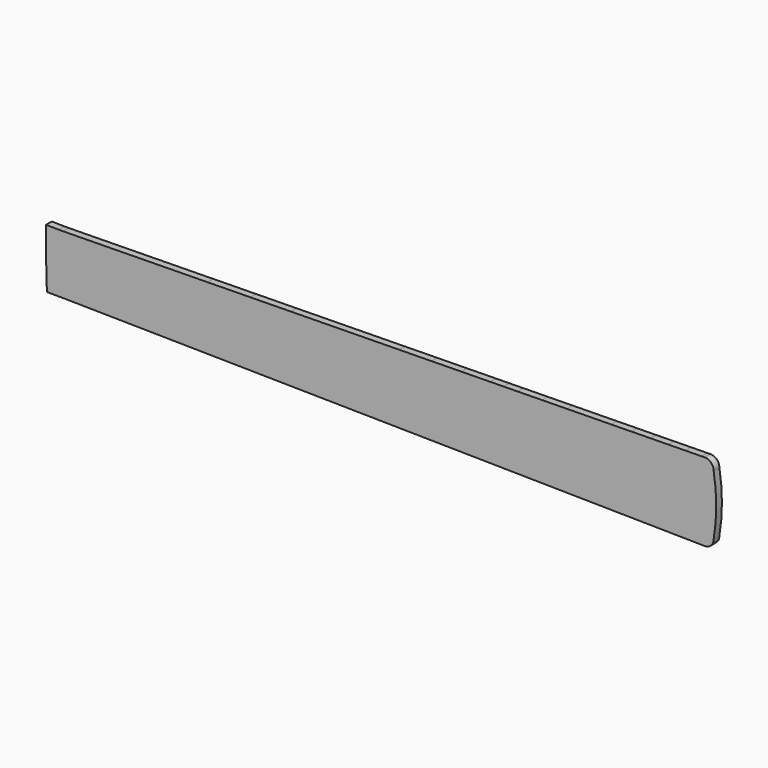
from build123d import *

# Parameters (mm, degrees)
F0_W     = 3.0600779591
F0_H     = 20.955
F1_DEPTH = 5.08


# Not quite as in the source:
# - a feature names something its author has since deleted; it is built from what else it names


with BuildPart() as f1:
    # F0 (on Front) → F1 (new body)
    with BuildSketch(Plane.XZ):
        with BuildLine():
            Line((211.1527612069, 54.1871569779), (194.9475612069, 53.9441942956))
            Line((194.9475612069, 53.9441942956), (194.9475612069, 27.6040292631))
            Line((194.9475612069, 27.6040292631), (199.8751612069, 27.6040292631))
            ThreePointArc((199.8751612069, 27.6040292631), (203.0501612069, 30.7790292631), (206.2251612069, 27.6040292631))
            Line((206.2251612069, 27.6040292631), (211.1527612069, 27.6040292631))
            Line((211.1527612069, 27.6040292631), (211.1527612069, 54.1871569779))
        make_face()
        with BuildLine():
            Line((35.1561612069, 27.6040292631), (25.4787612069, 27.6040292631))
            Line((25.4787612069, 27.6040292631), (25.4787612069, 3.8046848733))
            Line((25.4787612069, 3.8046848733), (51.1835612069, 3.4192950591))
            Line((51.1835612069, 3.4192950591), (51.1835612069, 27.6040292631))
            Line((51.1835612069, 27.6040292631), (41.5061612069, 27.6040292631))
            ThreePointArc((41.5061612069, 27.6040292631), (38.3311612069, 24.4290292631), (35.1561612069, 27.6040292631))
        make_face()
        Polygon((75.4405612069, 52.1524397183), (51.1835612069, 51.7887573333), (51.1835612069, 27.6040292631), (75.4405612069, 27.6040292631), align=None)
        Polygon((119.9667612069, 52.8200158658), (98.3513612069, 52.4959386829), (98.3513612069, 27.6040292631), (119.9667612069, 27.6040292631), align=None)
        Polygon((-127.8864387931, 6.1040758796), (-93.5710387931, 5.589588094), (-93.5710387931, 27.6040292631), (-127.8864387931, 27.6040292631), align=None)
        with BuildLine():
            ThreePointArc((-19.3522387931, 27.6040292631), (-16.1772387931, 30.7790292631), (-13.0022387931, 27.6040292631))
            Line((-13.0022387931, 27.6040292631), (-1.7500387931, 27.6040292631))
            Line((-1.7500387931, 27.6040292631), (-1.7500387931, 50.9951300136))
            Line((-1.7500387931, 50.9951300136), (-30.6044387931, 50.5625193442))
            Line((-30.6044387931, 50.5625193442), (-30.6044387931, 27.6040292631))
            Line((-30.6044387931, 27.6040292631), (-19.3522387931, 27.6040292631))
        make_face()
        Polygon((-93.5710387931, 27.6040292631), (-93.5710387931, 49.6184684202), (-127.8864387931, 49.1039816117), (-127.8864387931, 27.6040292631), align=None)
        Polygon((-30.6044387931, 4.6455353771), (-30.6044387931, 27.6040292631), (-61.1860387931, 27.6040292631), (-61.1860387931, 5.1040426264), align=None)
        Polygon((51.1835612069, 27.6040292631), (51.1835612069, 3.4192950591), (75.4405612069, 3.0556119834), (75.4405612069, 27.6040292631), align=None)
        Polygon((119.9667612069, 27.6040292631), (119.9667612069, 2.388034568), (140.3629612069, 2.0822361285), (140.3629612069, 14.6379053581), (140.3629612069, 27.6040292631), align=None)
        Polygon((98.3513612069, 27.6040292631), (98.3513612069, 2.7121123663), (119.9667612069, 2.388034568), (119.9667612069, 27.6040292631), align=None)
        with BuildLine():
            Line((-74.2035387931, 27.6040292631), (-61.1860387931, 27.6040292631))
            Line((-61.1860387931, 27.6040292631), (-61.1860387931, 50.1040129656))
            Line((-61.1860387931, 50.1040129656), (-93.5710387931, 49.6184684202))
            Line((-93.5710387931, 49.6184684202), (-93.5710387931, 27.6040292631))
            Line((-93.5710387931, 27.6040292631), (-80.5535387931, 27.6040292631))
            ThreePointArc((-80.5535387931, 27.6040292631), (-77.3785387931, 30.7790292631), (-74.2035387931, 27.6040292631))
        make_face()
        with BuildLine():
            Line((25.4787612069, 51.403368251), (25.4787612069, 27.6040292631))
            Line((25.4787612069, 27.6040292631), (35.1561612069, 27.6040292631))
            ThreePointArc((35.1561612069, 27.6040292631), (38.3311612069, 30.7790292631), (41.5061612069, 27.6040292631))
            Line((41.5061612069, 27.6040292631), (51.1835612069, 27.6040292631))
            Line((51.1835612069, 27.6040292631), (51.1835612069, 51.7887573333))
            Line((51.1835612069, 51.7887573333), (25.4787612069, 51.403368251))
        make_face()
        Polygon((-61.1860387931, 27.6040292631), (-30.6044387931, 27.6040292631), (-30.6044387931, 50.5625193442), (-61.1860387931, 50.1040129656), align=None)
        Polygon((-164.2338387931, 6.6490292631), (-127.8864387931, 6.1040758796), (-127.8864387931, 27.6040292631), (-164.2338387931, 27.6040292631), align=None)
        with BuildLine():
            Line((-167.2939167522, 27.6040292631), (-167.2939167522, 48.5590292631))
            add(Edge.make_bspline(
                [(-167.2939167522, 48.5590292631), (-169.3608924509, 48.5160966839), (-172.2759226046, 48.4555494006), (-175.4017391189, 48.6513352899), (-176.2988387931, 48.7219685213)],
                knots=[0, 0, 0, 0, 0.0767284167, 0.1082616947, 0.1082616947, 0.1082616947, 0.1082616947], degree=3))
            Line((-176.2988387931, 48.7219685213), (-176.2988387931, 27.6040292631))
            Line((-176.2988387931, 27.6040292631), (-167.2939167522, 27.6040292631))
        make_face()
        with BuildLine():
            Line((75.4405612069, 27.6040292631), (75.4405612069, 3.0556119834))
            Line((75.4405612069, 3.0556119834), (98.3513612069, 2.7121123663))
            Line((98.3513612069, 2.7121123663), (98.3513612069, 27.6040292631))
            Line((98.3513612069, 27.6040292631), (90.0709612069, 27.6040292631))
            ThreePointArc((90.0709612069, 27.6040292631), (86.8959612069, 24.4290292631), (83.7209612069, 27.6040292631))
            Line((83.7209612069, 27.6040292631), (75.4405612069, 27.6040292631))
        make_face()
        Polygon((177.2945612069, 27.6040292631), (177.2945612069, 1.5285238855), (194.9475612069, 1.2638540032), (194.9475612069, 27.6040292631), align=None)
        with BuildLine():
            Line((98.3513612069, 52.4959386829), (75.4405612069, 52.1524397183))
            Line((75.4405612069, 52.1524397183), (75.4405612069, 27.6040292631))
            Line((75.4405612069, 27.6040292631), (83.7209612069, 27.6040292631))
            ThreePointArc((83.7209612069, 27.6040292631), (86.8959612069, 30.7790292631), (90.0709612069, 27.6040292631))
            Line((90.0709612069, 27.6040292631), (98.3513612069, 27.6040292631))
            Line((98.3513612069, 27.6040292631), (98.3513612069, 52.4959386829))
        make_face()
        with BuildLine():
            Line((194.9475612069, 27.6040292631), (194.9475612069, 1.2638540032))
            Line((194.9475612069, 1.2638540032), (211.1527612069, 1.0208908594))
            Line((211.1527612069, 1.0208908594), (211.1527612069, 27.6040292631))
            Line((211.1527612069, 27.6040292631), (206.2251612069, 27.6040292631))
            ThreePointArc((206.2251612069, 27.6040292631), (203.0501612069, 24.4290292631), (199.8751612069, 27.6040292631))
            Line((199.8751612069, 27.6040292631), (194.9475612069, 27.6040292631))
        make_face()
        Polygon((-127.8864387931, 27.6040292631), (-127.8864387931, 49.1039816117), (-164.2338387931, 48.5590292631), (-164.2338387931, 27.6040292631), align=None)
        Polygon((140.3629612069, 53.1258137246), (119.9667612069, 52.8200158658), (119.9667612069, 27.6040292631), (140.3629612069, 27.6040292631), (140.3629612069, 40.5701442208), align=None)
        with BuildLine():
            Line((-1.7500387931, 27.6040292631), (-13.0022387931, 27.6040292631))
            ThreePointArc((-13.0022387931, 27.6040292631), (-16.1772387931, 24.4290292631), (-19.3522387931, 27.6040292631))
            Line((-19.3522387931, 27.6040292631), (-30.6044387931, 27.6040292631))
            Line((-30.6044387931, 27.6040292631), (-30.6044387931, 4.6455353771))
            Line((-30.6044387931, 4.6455353771), (-1.7500387931, 4.212923886))
            Line((-1.7500387931, 4.212923886), (-1.7500387931, 27.6040292631))
        make_face()
        Polygon((267.3121612069, 27.6040292631), (267.3121612069, 0.1788978957), (279.4533612069, -0.0031340521), (279.4533612069, 27.6040292631), align=None)
        Polygon((194.9475612069, 53.9441942956), (177.2945612069, 53.679524916), (177.2945612069, 27.6040292631), (194.9475612069, 27.6040292631), align=None)
        with BuildLine():
            Line((290.9087612069, 55.382929427), (279.4533612069, 55.2111799446))
            Line((279.4533612069, 55.2111799446), (279.4533612069, 27.6040292631))
            Line((279.4533612069, 27.6040292631), (282.0060612069, 27.6040292631))
            ThreePointArc((282.0060612069, 27.6040292631), (285.1810612069, 30.7790292631), (288.3560612069, 27.6040292631))
            Line((288.3560612069, 27.6040292631), (290.9087612069, 27.6040292631))
            Line((290.9087612069, 27.6040292631), (290.9087612069, 55.382929427))
        make_face()
        Polygon((279.4533612069, 55.2111799446), (267.3121612069, 55.0291483425), (267.3121612069, 27.6040292631), (279.4533612069, 27.6040292631), align=None)
        Polygon((177.2945612069, 53.679524916), (159.6161612069, 53.4144747171), (159.6161612069, 40.5701442208), (159.6161612069, 27.6040292631), (177.2945612069, 27.6040292631), align=None)
        with BuildLine():
            Line((140.3629612069, 14.6379053581), (140.3629612069, 2.0822361285))
            Line((140.3629612069, 2.0822361285), (149.9895612069, 1.9379053581))
            Line((149.9895612069, 1.9379053581), (149.9895612069, 11.4629053581))
            ThreePointArc((149.9895612069, 11.4629053581), (147.7444971767, 12.3928413278), (146.8145612069, 14.6379053581))
            Line((146.8145612069, 14.6379053581), (140.3629612069, 14.6379053581))
        make_face()
        with BuildLine():
            Line((226.4181612069, 27.6040292631), (226.4181612069, 0.7920180547))
            Line((226.4181612069, 0.7920180547), (240.8453612069, 0.5757123092))
            Line((240.8453612069, 0.5757123092), (240.8453612069, 27.6040292631))
            Line((240.8453612069, 27.6040292631), (236.8067612069, 27.6040292631))
            ThreePointArc((236.8067612069, 27.6040292631), (233.6317612069, 24.4290292631), (230.4567612069, 27.6040292631))
            Line((230.4567612069, 27.6040292631), (226.4181612069, 27.6040292631))
        make_face()
        Polygon((211.1527612069, 27.6040292631), (211.1527612069, 1.0208908594), (226.4181612069, 0.7920180547), (226.4181612069, 27.6040292631), align=None)
        Polygon((254.4597612069, 54.8364538014), (240.8453612069, 54.6323346827), (240.8453612069, 27.6040292631), (254.4597612069, 27.6040292631), align=None)
        Polygon((159.6161612069, 14.6379053581), (159.6161612069, 1.7935745878), (177.2945612069, 1.5285238855), (177.2945612069, 27.6040292631), (159.6161612069, 27.6040292631), align=None)
        with BuildLine():
            Line((267.3121612069, 55.0291483425), (254.4597612069, 54.8364538014))
            Line((254.4597612069, 54.8364538014), (254.4597612069, 27.6040292631))
            Line((254.4597612069, 27.6040292631), (257.7109612069, 27.6040292631))
            ThreePointArc((257.7109612069, 27.6040292631), (260.8859612069, 30.7790292631), (264.0609612069, 27.6040292631))
            Line((264.0609612069, 27.6040292631), (267.3121612069, 27.6040292631))
            Line((267.3121612069, 27.6040292631), (267.3121612069, 55.0291483425))
        make_face()
        with BuildLine():
            Line((149.9895612069, 53.2701442208), (140.3629612069, 53.1258137246))
            Line((140.3629612069, 53.1258137246), (140.3629612069, 40.5701442208))
            Line((140.3629612069, 40.5701442208), (146.8145612069, 40.5701442208))
            ThreePointArc((146.8145612069, 40.5701442208), (147.7444971767, 42.8152082511), (149.9895612069, 43.7451442208))
            Line((149.9895612069, 43.7451442208), (149.9895612069, 53.2701442208))
        make_face()
        with BuildLine():
            Line((240.8453612069, 54.6323346827), (226.4181612069, 54.4160293479))
            Line((226.4181612069, 54.4160293479), (226.4181612069, 27.6040292631))
            Line((226.4181612069, 27.6040292631), (230.4567612069, 27.6040292631))
            ThreePointArc((230.4567612069, 27.6040292631), (233.6317612069, 30.7790292631), (236.8067612069, 27.6040292631))
            Line((236.8067612069, 27.6040292631), (240.8453612069, 27.6040292631))
            Line((240.8453612069, 27.6040292631), (240.8453612069, 54.6323346827))
        make_face()
        Polygon((226.4181612069, 54.4160293479), (211.1527612069, 54.1871569779), (211.1527612069, 27.6040292631), (226.4181612069, 27.6040292631), align=None)
        Polygon((-1.7500387931, 50.9951300136), (-1.7500387931, 27.6040292631), (25.4787612069, 27.6040292631), (25.4787612069, 51.403368251), align=None)
        Polygon((25.4787612069, 27.6040292631), (-1.7500387931, 27.6040292631), (-1.7500387931, 4.212923886), (25.4787612069, 3.8046848733), align=None)
        Polygon((240.8453612069, 27.6040292631), (240.8453612069, 0.5757123092), (254.4597612069, 0.3715928028), (254.4597612069, 27.6040292631), align=None)
        with BuildLine():
            Line((-61.1860387931, 5.1040426264), (-61.1860387931, 27.6040292631))
            Line((-61.1860387931, 27.6040292631), (-74.2035387931, 27.6040292631))
            ThreePointArc((-74.2035387931, 27.6040292631), (-77.3785387931, 24.4290292631), (-80.5535387931, 27.6040292631))
            Line((-80.5535387931, 27.6040292631), (-93.5710387931, 27.6040292631))
            Line((-93.5710387931, 27.6040292631), (-93.5710387931, 5.589588094))
            Line((-93.5710387931, 5.589588094), (-61.1860387931, 5.1040426264))
        make_face()
        with BuildLine():
            Line((254.4597612069, 27.6040292631), (254.4597612069, 0.3715928028))
            Line((254.4597612069, 0.3715928028), (267.3121612069, 0.1788978957))
            Line((267.3121612069, 0.1788978957), (267.3121612069, 27.6040292631))
            Line((267.3121612069, 27.6040292631), (264.0609612069, 27.6040292631))
            ThreePointArc((264.0609612069, 27.6040292631), (260.8859612069, 24.4290292631), (257.7109612069, 27.6040292631))
            Line((257.7109612069, 27.6040292631), (254.4597612069, 27.6040292631))
        make_face()
        with BuildLine():
            ThreePointArc((41.5061612069, 27.6040292631), (38.3311612069, 30.7790292631), (35.1561612069, 27.6040292631))
            Line((35.1561612069, 27.6040292631), (41.5061612069, 27.6040292631))
        make_face()
        with BuildLine():
            Line((41.5061612069, 27.6040292631), (35.1561612069, 27.6040292631))
            ThreePointArc((35.1561612069, 27.6040292631), (38.3311612069, 24.4290292631), (41.5061612069, 27.6040292631))
        make_face()
        with BuildLine():
            ThreePointArc((90.0709612069, 27.6040292631), (86.8959612069, 30.7790292631), (83.7209612069, 27.6040292631))
            Line((83.7209612069, 27.6040292631), (90.0709612069, 27.6040292631))
        make_face()
        with BuildLine():
            Line((149.9895612069, 27.6040292631), (140.3629612069, 27.6040292631))
            Line((140.3629612069, 27.6040292631), (140.3629612069, 14.6379053581))
            Line((140.3629612069, 14.6379053581), (146.8145612069, 14.6379053581))
            ThreePointArc((146.8145612069, 14.6379053581), (147.7444971767, 16.8829693884), (149.9895612069, 17.8129053581))
            Line((149.9895612069, 17.8129053581), (149.9895612069, 27.6040292631))
        make_face()
        with BuildLine():
            Line((-80.5535387931, 27.6040292631), (-74.2035387931, 27.6040292631))
            ThreePointArc((-74.2035387931, 27.6040292631), (-77.3785387931, 30.7790292631), (-80.5535387931, 27.6040292631))
        make_face()
        with BuildLine():
            ThreePointArc((-80.5535387931, 27.6040292631), (-77.3785387931, 24.4290292631), (-74.2035387931, 27.6040292631))
            Line((-74.2035387931, 27.6040292631), (-80.5535387931, 27.6040292631))
        make_face()
        with BuildLine():
            Line((-19.3522387931, 27.6040292631), (-13.0022387931, 27.6040292631))
            ThreePointArc((-13.0022387931, 27.6040292631), (-16.1772387931, 30.7790292631), (-19.3522387931, 27.6040292631))
        make_face()
        with BuildLine():
            ThreePointArc((-19.3522387931, 27.6040292631), (-16.1772387931, 24.4290292631), (-13.0022387931, 27.6040292631))
            Line((-13.0022387931, 27.6040292631), (-19.3522387931, 27.6040292631))
        make_face()
        with BuildLine():
            Line((90.0709612069, 27.6040292631), (83.7209612069, 27.6040292631))
            ThreePointArc((83.7209612069, 27.6040292631), (86.8959612069, 24.4290292631), (90.0709612069, 27.6040292631))
        make_face()
        with BuildLine():
            Line((279.4533612069, 27.6040292631), (279.4533612069, -0.0031340521))
            Line((279.4533612069, -0.0031340521), (290.9087612069, -0.1748838606))
            Line((290.9087612069, -0.1748838606), (290.9087612069, 27.6040292631))
            Line((290.9087612069, 27.6040292631), (288.3560612069, 27.6040292631))
            ThreePointArc((288.3560612069, 27.6040292631), (285.1810612069, 24.4290292631), (282.0060612069, 27.6040292631))
            Line((282.0060612069, 27.6040292631), (279.4533612069, 27.6040292631))
        make_face()
        with BuildLine():
            Line((159.6161612069, 27.6040292631), (149.9895612069, 27.6040292631))
            Line((149.9895612069, 27.6040292631), (149.9895612069, 17.8129053581))
            ThreePointArc((149.9895612069, 17.8129053581), (152.2346252372, 16.8829693884), (153.1645612069, 14.6379053581))
            Line((153.1645612069, 14.6379053581), (159.6161612069, 14.6379053581))
            Line((159.6161612069, 14.6379053581), (159.6161612069, 27.6040292631))
        make_face()
        with BuildLine():
            ThreePointArc((299.5327314187, 49.000836976), (297.6965766308, 53.53366288), (293.1831626072, 55.4170292631))
            Line((293.1831626072, 55.4170292631), (293.1827280197, 27.6040292631))
            Line((293.1827280197, 27.6040292631), (293.1822934321, -0.2089707301))
            ThreePointArc((293.1822934321, -0.2089707301), (297.6944667131, 1.6729676451), (299.5320740528, 6.2033759083))
            ThreePointArc((299.5320740528, 6.2033759083), (301.3481611896, 27.6020785522), (299.5327314187, 49.000836976))
        make_face()
        with BuildLine():
            Line((146.8145612069, 40.5701442208), (140.3629612069, 40.5701442208))
            Line((140.3629612069, 40.5701442208), (140.3629612069, 27.6040292631))
            Line((140.3629612069, 27.6040292631), (149.9895612069, 27.6040292631))
            Line((149.9895612069, 27.6040292631), (149.9895612069, 37.3951442208))
            ThreePointArc((149.9895612069, 37.3951442208), (147.7444971767, 38.3250801906), (146.8145612069, 40.5701442208))
        make_face()
        with BuildLine():
            Line((149.9895612069, 37.3951442208), (149.9895612069, 27.6040292631))
            Line((149.9895612069, 27.6040292631), (159.6161612069, 27.6040292631))
            Line((159.6161612069, 27.6040292631), (159.6161612069, 40.5701442208))
            Line((159.6161612069, 40.5701442208), (153.1645612069, 40.5701442208))
            ThreePointArc((153.1645612069, 40.5701442208), (152.2346252372, 38.3250801906), (149.9895612069, 37.3951442208))
        make_face()
        with BuildLine():
            Line((149.9895612069, 11.4629053581), (149.9895612069, 1.9379053581))
            Line((149.9895612069, 1.9379053581), (159.6161612069, 1.7935745878))
            Line((159.6161612069, 1.7935745878), (159.6161612069, 14.6379053581))
            Line((159.6161612069, 14.6379053581), (153.1645612069, 14.6379053581))
            ThreePointArc((153.1645612069, 14.6379053581), (152.2346252372, 12.3928413278), (149.9895612069, 11.4629053581))
        make_face()
        with BuildLine():
            Line((159.6161612069, 53.4144747171), (149.9895612069, 53.2701442208))
            Line((149.9895612069, 53.2701442208), (149.9895612069, 43.7451442208))
            ThreePointArc((149.9895612069, 43.7451442208), (152.2346252372, 42.8152082511), (153.1645612069, 40.5701442208))
            Line((153.1645612069, 40.5701442208), (159.6161612069, 40.5701442208))
            Line((159.6161612069, 40.5701442208), (159.6161612069, 53.4144747171))
        make_face()
        with BuildLine():
            ThreePointArc((149.9895612069, 17.8129053581), (147.7444971767, 16.8829693884), (146.8145612069, 14.6379053581))
            Line((146.8145612069, 14.6379053581), (149.9895612069, 14.6379053581))
            Line((149.9895612069, 14.6379053581), (149.9895612069, 17.8129053581))
        make_face()
        with BuildLine():
            Line((149.9895612069, 40.5701442208), (149.9895612069, 43.7451442208))
            ThreePointArc((149.9895612069, 43.7451442208), (147.7444971767, 42.8152082511), (146.8145612069, 40.5701442208))
            Line((146.8145612069, 40.5701442208), (149.9895612069, 40.5701442208))
        make_face()
        with BuildLine():
            Line((206.2251612069, 27.6040292631), (199.8751612069, 27.6040292631))
            ThreePointArc((199.8751612069, 27.6040292631), (203.0501612069, 24.4290292631), (206.2251612069, 27.6040292631))
        make_face()
        with BuildLine():
            ThreePointArc((206.2251612069, 27.6040292631), (203.0501612069, 30.7790292631), (199.8751612069, 27.6040292631))
            Line((199.8751612069, 27.6040292631), (206.2251612069, 27.6040292631))
        make_face()
        with BuildLine():
            ThreePointArc((236.8067612069, 27.6040292631), (233.6317612069, 30.7790292631), (230.4567612069, 27.6040292631))
            Line((230.4567612069, 27.6040292631), (236.8067612069, 27.6040292631))
        make_face()
        with BuildLine():
            ThreePointArc((288.3560612069, 27.6040292631), (285.1810612069, 30.7790292631), (282.0060612069, 27.6040292631))
            Line((282.0060612069, 27.6040292631), (288.3560612069, 27.6040292631))
        make_face()
        with BuildLine():
            Line((236.8067612069, 27.6040292631), (230.4567612069, 27.6040292631))
            ThreePointArc((230.4567612069, 27.6040292631), (233.6317612069, 24.4290292631), (236.8067612069, 27.6040292631))
        make_face()
        with BuildLine():
            ThreePointArc((264.0609612069, 27.6040292631), (260.8859612069, 30.7790292631), (257.7109612069, 27.6040292631))
            Line((257.7109612069, 27.6040292631), (264.0609612069, 27.6040292631))
        make_face()
        with BuildLine():
            Line((264.0609612069, 27.6040292631), (257.7109612069, 27.6040292631))
            ThreePointArc((257.7109612069, 27.6040292631), (260.8859612069, 24.4290292631), (264.0609612069, 27.6040292631))
        make_face()
        with BuildLine():
            Line((288.3560612069, 27.6040292631), (282.0060612069, 27.6040292631))
            ThreePointArc((282.0060612069, 27.6040292631), (285.1810612069, 24.4290292631), (288.3560612069, 27.6040292631))
        make_face()
        Polygon((290.9087612069, 27.6040292631), (290.9087612069, -0.1748838606), (293.1822934321, -0.2089707301), (293.1827280197, 27.6040292631), align=None)
        with BuildLine():
            ThreePointArc((153.1645612069, 14.6379053581), (152.2346252372, 16.8829693884), (149.9895612069, 17.8129053581))
            Line((149.9895612069, 17.8129053581), (149.9895612069, 14.6379053581))
            Line((149.9895612069, 14.6379053581), (153.1645612069, 14.6379053581))
        make_face()
        with BuildLine():
            ThreePointArc((146.8145612069, 14.6379053581), (147.7444971767, 12.3928413278), (149.9895612069, 11.4629053581))
            Line((149.9895612069, 11.4629053581), (149.9895612069, 14.6379053581))
            Line((149.9895612069, 14.6379053581), (146.8145612069, 14.6379053581))
        make_face()
        Polygon((293.1831626072, 55.4170292631), (290.9087612069, 55.382929427), (290.9087612069, 27.6040292631), (293.1827280197, 27.6040292631), align=None)
        with BuildLine():
            ThreePointArc((149.9895612069, 37.3951442208), (152.2346252372, 38.3250801906), (153.1645612069, 40.5701442208))
            Line((153.1645612069, 40.5701442208), (149.9895612069, 40.5701442208))
            Line((149.9895612069, 40.5701442208), (149.9895612069, 37.3951442208))
        make_face()
        with Locations((-165.7638777726, 38.0815292631)):
            Rectangle(F0_W, F0_H)
        with Locations((-165.7638777726, 17.1265292631)):
            Rectangle(F0_W, F0_H)
        with BuildLine():
            Line((149.9895612069, 14.6379053581), (149.9895612069, 11.4629053581))
            ThreePointArc((149.9895612069, 11.4629053581), (152.2346252372, 12.3928413278), (153.1645612069, 14.6379053581))
            Line((153.1645612069, 14.6379053581), (149.9895612069, 14.6379053581))
        make_face()
        with BuildLine():
            Line((149.9895612069, 40.5701442208), (146.8145612069, 40.5701442208))
            ThreePointArc((146.8145612069, 40.5701442208), (147.7444971767, 38.3250801906), (149.9895612069, 37.3951442208))
            Line((149.9895612069, 37.3951442208), (149.9895612069, 40.5701442208))
        make_face()
        with BuildLine():
            ThreePointArc((153.1645612069, 40.5701442208), (152.2346252372, 42.8152082511), (149.9895612069, 43.7451442208))
            Line((149.9895612069, 43.7451442208), (149.9895612069, 40.5701442208))
            Line((149.9895612069, 40.5701442208), (153.1645612069, 40.5701442208))
        make_face()
        Polygon((-175.7287366174, 6.6946032245), (-167.2939167522, 6.6490292631), (-167.2939167522, 27.6040292631), (-176.2988387931, 27.6040292631), align=None)
    extrude(amount=-F1_DEPTH)


solid = f1.part
